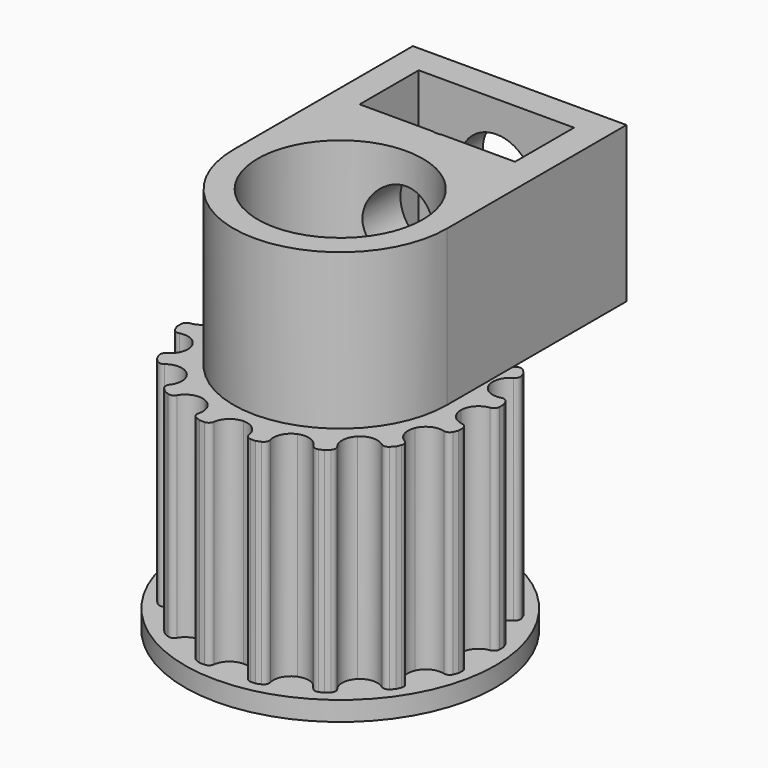
from build123d import *

# Parameters (mm, degrees)
F0_R             = 7.6394373987
F0_R_2           = 4.25
F1_DEPTH         = 11
F3_DEPTH         = 11.001
F3_COPIES_COUNT  = 8
F3_COPIES_ANGLE  = 157.5
F3_COPIES1_COUNT = 9
F3_COPIES1_ANGLE = 180
F4_R             = 8
F4_R_2           = 4.25
F5_DEPTH         = 1
F6_R             = 4.25
F7_DEPTH         = 8
F8_R             = 1.9
F9_DEPTH         = 10


# Not quite as in the source:
# - ends of sketch curves that miss each other by under 0.0002 mm in the source are joined
# - a pattern or mirror of a feature is missing from the dataset's text; its kind, count and spacing are read off the source's solid
# - a feature names something its author has since deleted; it is built from what else it names


with BuildPart() as f1:
    # F0 (on Top) → F1 (new body)
    with BuildSketch(Plane.XY):
        Circle(F0_R)
        Circle(F0_R_2, mode=Mode.SUBTRACT)
    extrude(amount=F1_DEPTH)

    # F2 (on Top) → F3 (cut, through all)
    with BuildSketch(Plane.XY):
        with BuildLine():
            ThreePointArc((0.9017719181, -7.0023415032), (0.5987456618, -6.4391610804), (0, -6.2144373987))
            ThreePointArc((0, -6.2144373987), (-0.5987456618, -6.4391610804), (-0.9017719181, -7.0023415032))
            ThreePointArc((-0.9017719181, -7.0023415032), (-0.9975198669, -7.184187159), (-1.1896796808, -7.25699))
            Line((-1.1896796808, -7.25699), (-2.3868598428, -7.25699))
            ThreePointArc((-2.3868598428, -7.25699), (0, -7.6394373987), (2.3868598428, -7.25699))
            Line((2.3868598428, -7.25699), (1.1896796808, -7.25699))
            ThreePointArc((1.1896796808, -7.25699), (0.9975198669, -7.184187159), (0.9017719181, -7.0023415032))
        make_face()
    f3 = extrude(amount=F3_DEPTH, mode=Mode.SUBTRACT)

    # F3_copies: F3 ×8 about axis
    f3_copies_axis = Axis((0, 0, 0), (0, 0, -1))
    for i in range(1, F3_COPIES_COUNT):
        add(f3.rotate(f3_copies_axis, i * F3_COPIES_ANGLE / (F3_COPIES_COUNT - 1)), mode=Mode.SUBTRACT)

    # F3_copies1: F3 ×9 about axis
    f3_copies1_axis = Axis((0, 0, 0), (0, 0, 1))
    for i in range(1, F3_COPIES1_COUNT):
        add(f3.rotate(f3_copies1_axis, i * F3_COPIES1_ANGLE / (F3_COPIES1_COUNT - 1)), mode=Mode.SUBTRACT)

    # F4 (on face) → F5 (join)
    with BuildSketch(Plane(origin=(0, 0, 0), x_dir=(1, 0, 0), z_dir=(0, 0, -1))):
        Circle(F4_R)
        Circle(F4_R_2, mode=Mode.SUBTRACT)
    extrude(amount=F5_DEPTH)

    # F6 (on face) → F7 (join)
    with BuildSketch(Plane.XY.offset(11)):
        with BuildLine():
            Line((-5.5, 4.2538924505), (-5.5, 0))
            ThreePointArc((-5.5, 0), (0, -5.5), (5.5, 0))
            Line((5.5, 0), (5.5, 4.2538924505))
            ThreePointArc((5.5, 4.2538924505), (4.3574531497, 4.4333271044), (4.3137541227, 5.5890521994))
            ThreePointArc((4.3137541227, 5.5890521994), (4.3746351807, 5.7853277116), (4.2902362702, 5.9726974098))
            Line((4.2902362702, 5.9726974098), (4.1107546227, 6.1521790573))
            Line((4.1107546227, 6.1521790573), (3.8762505492, 6.249313825))
            ThreePointArc((3.8762505492, 6.249313825), (3.8754150111, 6.2496582146), (3.8745784043, 6.25))
            Line((3.8745784043, 6.25), (3.6559571933, 6.25))
            ThreePointArc((3.6559571933, 6.25), (3.5737630913, 6.1992003777), (3.5128086992, 6.1242268216))
            ThreePointArc((3.5128086992, 6.1242268216), (2.65655008, 5.6748069492), (1.8791762967, 6.25))
            Line((1.8791762967, 6.25), (0.2519111663, 6.25))
            ThreePointArc((0.2519111663, 6.25), (0, 6.2144373987), (-0.2519111663, 6.25))
            Line((-0.2519111663, 6.25), (-1.8791762967, 6.25))
            ThreePointArc((-1.8791762967, 6.25), (-2.65655008, 5.6748069492), (-3.5128086992, 6.1242268216))
            ThreePointArc((-3.5128086992, 6.1242268216), (-3.5737630913, 6.1992003777), (-3.6559571933, 6.25))
            Line((-3.6559571933, 6.25), (-3.8745784043, 6.25))
            ThreePointArc((-3.8745784043, 6.25), (-3.8754150111, 6.2496582146), (-3.8762505492, 6.249313825))
            Line((-3.8762505492, 6.249313825), (-4.1107546227, 6.1521790573))
            Line((-4.1107546227, 6.1521790573), (-4.2902362702, 5.9726974098))
            ThreePointArc((-4.2902362702, 5.9726974098), (-4.3746351807, 5.7853277116), (-4.3137541227, 5.5890521994))
            ThreePointArc((-4.3137541227, 5.5890521994), (-4.3574531497, 4.4333271044), (-5.5, 4.2538924505))
        make_face()
        Circle(F6_R, mode=Mode.SUBTRACT)
        with BuildLine():
            Line((-5.5, 11.55), (-5.5, 4.2538924505))
            ThreePointArc((-5.5, 4.2538924505), (-4.3574531497, 4.4333271044), (-4.3137541227, 5.5890521994))
            ThreePointArc((-4.3137541227, 5.5890521994), (-4.3746351807, 5.7853277116), (-4.2902362702, 5.9726974098))
            Line((-4.2902362702, 5.9726974098), (-4.1107546227, 6.1521790573))
            Line((-4.1107546227, 6.1521790573), (-3.8762505492, 6.249313825))
            ThreePointArc((-3.8762505492, 6.249313825), (-3.8754150111, 6.2496582146), (-3.8745784043, 6.25))
            Line((-3.8745784043, 6.25), (-4, 6.25))
            Line((-4, 6.25), (-4, 10.05))
            Line((-4, 10.05), (4, 10.05))
            Line((4, 10.05), (4, 6.25))
            Line((4, 6.25), (3.8745784043, 6.25))
            ThreePointArc((3.8745784043, 6.25), (3.8754150111, 6.2496582146), (3.8762505492, 6.249313825))
            Line((3.8762505492, 6.249313825), (4.1107546227, 6.1521790573))
            Line((4.1107546227, 6.1521790573), (4.2902362702, 5.9726974098))
            ThreePointArc((4.2902362702, 5.9726974098), (4.3746351807, 5.7853277116), (4.3137541227, 5.5890521994))
            ThreePointArc((4.3137541227, 5.5890521994), (4.3574531497, 4.4333271044), (5.5, 4.2538924505))
            Line((5.5, 4.2538924505), (5.5, 11.55))
            Line((5.5, 11.55), (-5.5, 11.55))
        make_face()
        with BuildLine():
            Line((-1.8791762967, 6.25), (-3.6559571933, 6.25))
            ThreePointArc((-3.6559571933, 6.25), (-3.5737630913, 6.1992003777), (-3.5128086992, 6.1242268216))
            ThreePointArc((-3.5128086992, 6.1242268216), (-2.65655008, 5.6748069492), (-1.8791762967, 6.25))
        make_face()
        with BuildLine():
            ThreePointArc((3.5128086992, 6.1242268216), (3.5737630913, 6.1992003777), (3.6559571933, 6.25))
            Line((3.6559571933, 6.25), (1.8791762967, 6.25))
            ThreePointArc((1.8791762967, 6.25), (2.65655008, 5.6748069492), (3.5128086992, 6.1242268216))
        make_face()
    extrude(amount=F7_DEPTH)

    # F8 (on face) → F9 (cut)
    with BuildSketch(Plane(origin=(0, 11.55, 0), x_dir=(-1, 0, 0), z_dir=(0, 1, 0))):
        with Locations((0, 15.5)):
            Circle(F8_R)
    extrude(amount=-F9_DEPTH, mode=Mode.SUBTRACT)


solid = f1.part
